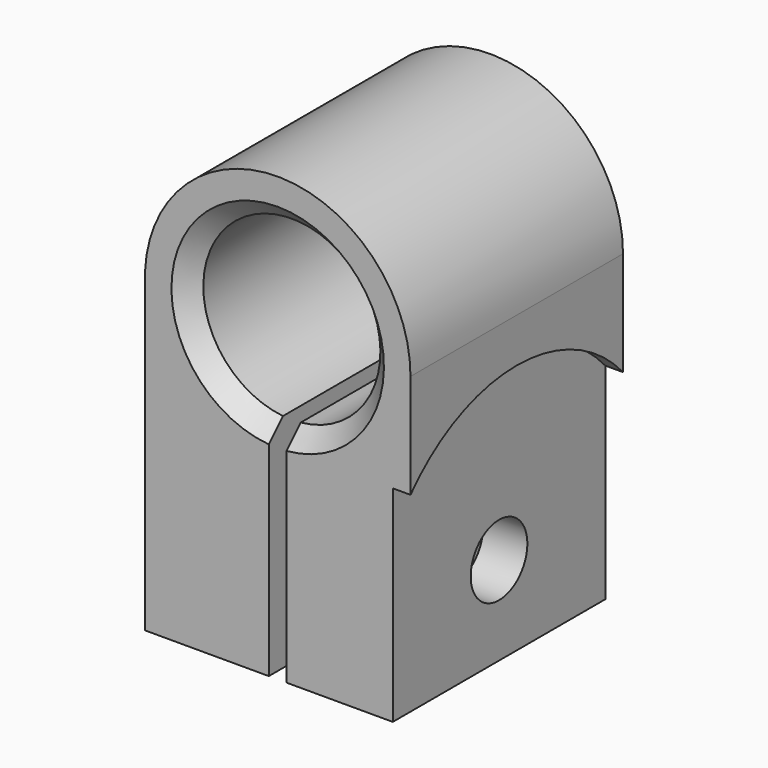
from build123d import *

# Parameters (mm, degrees)
F1_DEPTH  = 30
F2_R      = 10
F3_DEPTH  = 30.001
F5_DEPTH  = 30.001
F7_DEPTH  = 2
F8_R      = 4
F9_DEPTH  = 5
F10_SIZE2 = 2
F10_SIZE  = 2


with BuildPart() as f1:
    # F0 (on Front) → F1 (new body)
    with BuildSketch(Plane.XZ):
        with BuildLine():
            Line((-14.9850390488, 11.2684052181), (-14.9850390488, -24.4013743764))
            Line((-14.9850390488, -24.4013743764), (-0.9850390488, -24.4013743764))
            Line((-0.9850390488, -24.4013743764), (1, -24.4013743764))
            Line((1, -24.4013743764), (15, -24.4013743764))
            Line((15, -24.4013743764), (15, 10.5986256236))
            ThreePointArc((15, 10.5986256236), (0.334973333, 25.5948849194), (-14.9850390488, 11.2684052181))
        make_face()
    extrude(amount=F1_DEPTH)

    # F2 (on face) → F3 (cut, through all)
    with BuildSketch(Plane.XZ.offset(30)):
        with Locations((0, 10.5986256236)):
            Circle(F2_R)
    extrude(amount=-F3_DEPTH, mode=Mode.SUBTRACT)

    # F4 (on face) → F5 (cut, through all)
    with BuildSketch(Plane.XZ.offset(30)):
        with BuildLine():
            Line((-1, -24.4013743764), (0, -24.4013743764))
            Line((0, -24.4013743764), (1, -24.4013743764))
            Line((1, -24.4013743764), (1, 0.6487512526))
            ThreePointArc((1, 0.6487512526), (0, 0.5986256236), (-1, 0.6487512526))
            Line((-1, 0.6487512526), (-1, -24.4013743764))
        make_face()
    extrude(amount=-F5_DEPTH, mode=Mode.SUBTRACT)

    # F6 (on face) → F7 (cut)
    with BuildSketch(Plane.YZ.offset(15)):
        with BuildLine():
            Line((0, -24.4013743764), (0, -1.172617821))
            ThreePointArc((0, -1.172617821), (-15, 5.5986256236), (-30, -1.172617821))
            Line((-30, -1.172617821), (-30, -24.4013743764))
            Line((-30, -24.4013743764), (0, -24.4013743764))
        make_face()
    extrude(amount=-F7_DEPTH, mode=Mode.SUBTRACT)

    # F8 (on face) → F9 (cut, symmetric)
    with BuildSketch(Plane.YZ.offset(13)):
        with Locations((-15, -14.4013743764)):
            Circle(F8_R)
    extrude(amount=F9_DEPTH, both=True, mode=Mode.SUBTRACT)

    # F10
    f10_edges = [f1.edges().sort_by_distance(p)[0] for p in [
        (0, -30, 20.598626),
        (0, 0, 20.598626),
    ]]
    chamfer(f10_edges, length=F10_SIZE, length2=F10_SIZE2)


solid = f1.part
